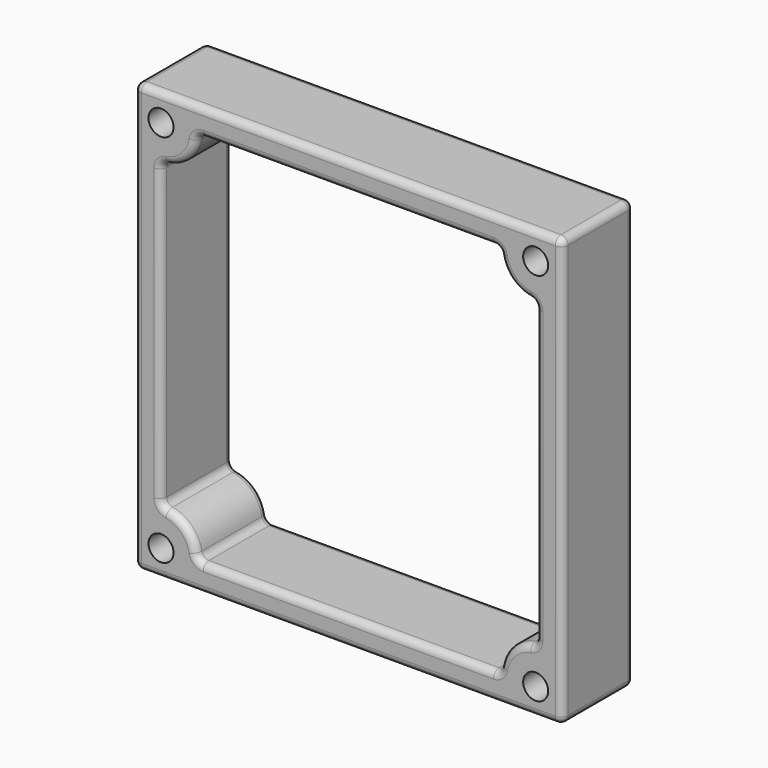
from build123d import *

# Parameters (mm, degrees)
F0_W     = 120
F0_H     = 120
F1_DEPTH = 25
F2_R     = 3.5
F3_DEPTH = 25
F5_DEPTH = 25
F6_F1_R  = 2
F6_F2_R  = 2


with BuildPart() as f1:
    # F0 (on Front) → F1 (new body)
    with BuildSketch(Plane.XZ):
        Rectangle(F0_W, F0_H)
    extrude(amount=F1_DEPTH)

    # F2 (on face) → F3 (cut)
    with BuildSketch(Plane.XZ.offset(25)):
        with Locations((-52.5, 52.5)):
            Circle(F2_R)
        with Locations((-52.5, -52.5)):
            Circle(F2_R)
        with Locations((52.5, -52.5)):
            Circle(F2_R)
        with Locations((52.5, 52.5)):
            Circle(F2_R)
    extrude(amount=-F3_DEPTH, mode=Mode.SUBTRACT)

    # F4 (on face) → F5 (cut)
    with BuildSketch(Plane.XZ.offset(25)):
        with BuildLine():
            ThreePointArc((52.5, 42.5), (45.4289321881, 45.4289321881), (42.5, 52.5))
            Line((42.5, 52.5), (-42.5, 52.5))
            ThreePointArc((-42.5, 52.5), (-45.4289321881, 45.4289321881), (-52.5, 42.5))
            Line((-52.5, 42.5), (-52.5, -42.5))
            ThreePointArc((-52.5, -42.5), (-45.4289321881, -45.4289321881), (-42.5, -52.5))
            Line((-42.5, -52.5), (42.5, -52.5))
            ThreePointArc((42.5, -52.5), (45.4289321881, -45.4289321881), (52.5, -42.5))
            Line((52.5, -42.5), (52.5, 42.5))
        make_face()
    extrude(amount=-F5_DEPTH, mode=Mode.SUBTRACT)

    # F6: fillet of radius 2 on 28 edges, made by hand

    # F6_f1
    f6_f1_edges = [f1.edges().sort_by_distance(p)[0] for p in [
        (42.5, -12.5, 52.5),
        (-42.5, -12.5, 52.5),
        (-52.5, -12.5, 42.5),
        (-52.5, -12.5, -42.5),
        (52.5, -12.5, -42.5),
        (52.5, -12.5, 42.5),
        (-42.5, -12.5, -52.5),
        (42.5, -12.5, -52.5),
    ]]
    fillet(f6_f1_edges, radius=F6_F1_R)

    # F6_f2
    f6_f2_edges = [f1.edges().sort_by_distance(p)[0] for p in [
        (-60, -12.5, 60),
        (-60, -12.5, -60),
        (-60, 0, 0),
        (-60, -25, 0),
        (60, -12.5, 60),
        (0, 0, 60),
        (0, -25, 60),
        (60, -12.5, -60),
        (60, 0, 0),
        (60, -25, 0),
        (0, 0, -60),
        (0, -25, -60),
        (0, -25, 52.5),
        (0, 0, 52.5),
        (-52.5, -25, 0),
        (-52.5, 0, 0),
        (52.5, -25, 0),
        (52.5, 0, 0),
        (0, -25, -52.5),
        (0, 0, -52.5),
        (-41.9588348825, 0, -52.0275252317),
        (41.9588348825, 0, -52.0275252317),
        (-41.9588348825, -25, -52.0275252317),
        (41.9588348825, -25, -52.0275252317),
        (52.0275252317, 0, -41.9588348825),
        (52.0275252317, 0, 41.9588348825),
        (52.0275252317, -25, -41.9588348825),
        (52.0275252317, -25, 41.9588348825),
        (-52.0275252317, 0, 41.9588348825),
        (-52.0275252317, 0, -41.9588348825),
        (-52.0275252317, -25, 41.9588348825),
        (-52.0275252317, -25, -41.9588348825),
        (41.9588348825, 0, 52.0275252317),
        (-41.9588348825, 0, 52.0275252317),
        (41.9588348825, -25, 52.0275252317),
        (-41.9588348825, -25, 52.0275252317),
    ]]
    fillet(f6_f2_edges, radius=F6_F2_R)


solid = f1.part
